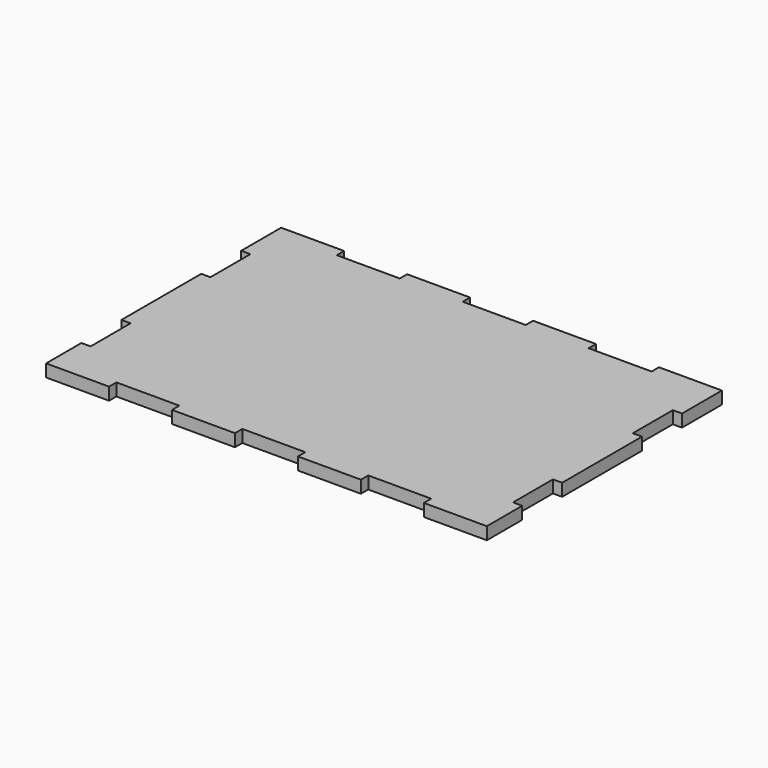
from build123d import *

# Parameters (mm, degrees)
F0_W     = 3.175
F0_H     = 14.0914226329
F0_H_2   = 17.2664226329
F0_H_3   = 12.0928868353
F0_W_2   = 18.5964285714
F0_H_4   = 3.175
F0_W_3   = 21.7714285714
F1_DEPTH = 4.29735


with BuildPart() as f1:
    # F0 (on Top) → F1 (new body)
    with BuildSketch(Plane.XY):
        with Locations((74.6125, 40.5792886835)):
            Rectangle(F0_W, F0_H)
        with Locations((74.6125, 7.6339434177)):
            Rectangle(F0_W, F0_H_2)
        with Locations((74.6125, -9.6324792153)):
            Rectangle(F0_W, F0_H_2)
        with Locations((74.6125, -41.5785565823)):
            Rectangle(F0_W, F0_H_3)
        with Locations((63.7267857143, -49.2125)):
            Rectangle(F0_W_2, F0_H_4)
        with Locations((21.7714285714, -49.2125)):
            Rectangle(F0_W_3, F0_H_4)
        with Locations((-21.7714285714, -49.2125)):
            Rectangle(F0_W_3, F0_H_4)
        with Locations((-63.7267857143, -49.2125)):
            Rectangle(F0_W_2, F0_H_4)
        with Locations((-74.6125, -41.5785565823)):
            Rectangle(F0_W, F0_H_3)
        with Locations((-74.6125, -9.6324792153)):
            Rectangle(F0_W, F0_H_2)
        with Locations((-74.6125, 7.6339434177)):
            Rectangle(F0_W, F0_H_2)
        with Locations((-74.6125, 40.5792886835)):
            Rectangle(F0_W, F0_H)
        with Locations((-63.7267857143, 49.2125)):
            Rectangle(F0_W_2, F0_H_4)
        with Locations((-21.7714285714, 49.2125)):
            Rectangle(F0_W_3, F0_H_4)
        with Locations((21.7714285714, 49.2125)):
            Rectangle(F0_W_3, F0_H_4)
        with Locations((63.7267857143, 49.2125)):
            Rectangle(F0_W_2, F0_H_4)
        Polygon((54.4285714286, -47.625), (73.025, -47.625), (73.025, -35.5321131647), (73.025, -18.2656905317), (73.025, -0.9992678988), (73.025, 16.2671547341), (73.025, 33.5335773671), (73.025, 47.625), (54.4285714286, 47.625), (32.6571428571, 47.625), (10.8857142857, 47.625), (-10.8857142857, 47.625), (-32.6571428571, 47.625), (-54.4285714286, 47.625), (-73.025, 47.625), (-73.025, 33.5335773671), (-73.025, 16.2671547341), (-73.025, -0.9992678988), (-73.025, -18.2656905317), (-73.025, -35.5321131647), (-73.025, -47.625), (-54.4285714286, -47.625), (-32.6571428571, -47.625), (-10.8857142857, -47.625), (10.8857142857, -47.625), (32.6571428571, -47.625), align=None)
        with Locations((74.6125, 49.2125)):
            Rectangle(F0_W, F0_H_4)
        with Locations((74.6125, -49.2125)):
            Rectangle(F0_W, F0_H_4)
        with Locations((-74.6125, -49.2125)):
            Rectangle(F0_W, F0_H_4)
        with Locations((-74.6125, 49.2125)):
            Rectangle(F0_W, F0_H_4)
    extrude(amount=-F1_DEPTH)


solid = f1.part
